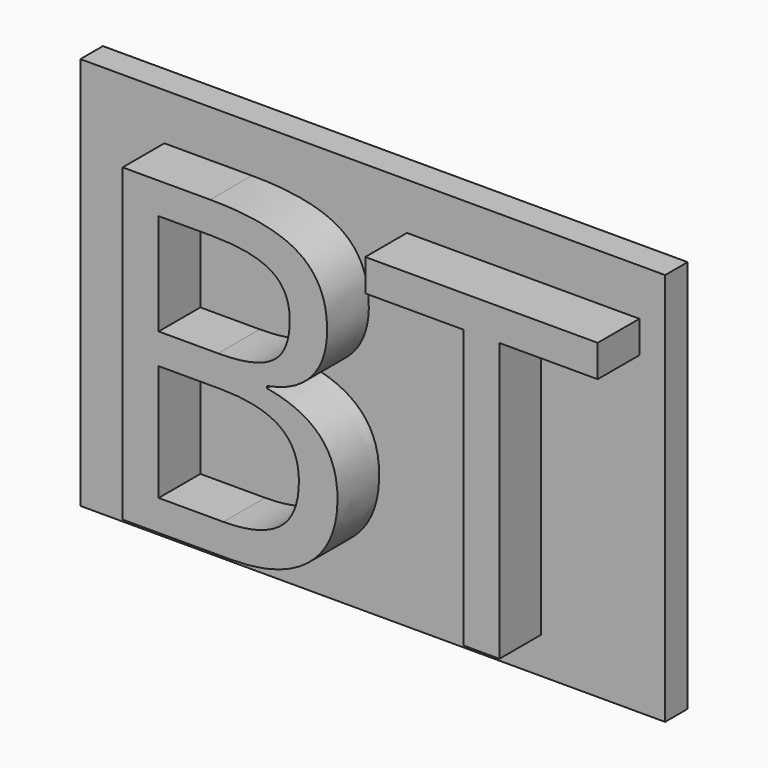
from build123d import *

# Parameters (mm, degrees)
F0_TEXT_SIZE = 105.8333333333
F1_DEPTH     = 12.7
F2_W         = 142.4835696816
F2_H         = 95.8525761962
F3_DEPTH     = 6.858


# Not quite as in the source:
# - Text() gives the source's letters only with a copy of the font that has no kerning and outlines rounded to 1/6400 em; it was checked with that copy


with BuildPart() as f1:
    # F0 (on Front) → F1 (new body)
    with BuildSketch(Plane.XZ):
        with Locations((-61.0680826703, -36.7489363135)):
            Text('BT', F0_TEXT_SIZE, font='Open Sans', text_align=(TextAlign.LEFT, TextAlign.BOTTOM))
    extrude(amount=F1_DEPTH)

    # F2 (on Front) → F3 (join)
    with BuildSketch(Plane.XZ):
        with Locations((0.0996403396, 2.2916942835)):
            Rectangle(F2_W, F2_H)
    extrude(amount=-F3_DEPTH)


solid = f1.part
